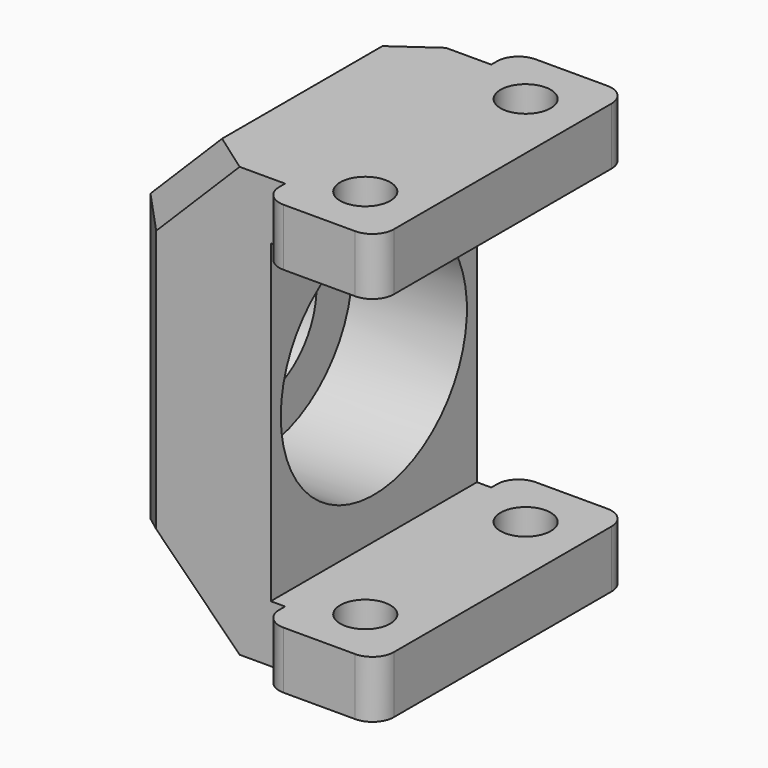
from build123d import *

# Parameters (mm, degrees)
F2_R      = 3
F2_W      = 1
F2_H      = 18
F3_DEPTH  = 4
F4_START  = 2
F2_R_2    = 1.75
F4_DEPTH  = 2
F2_W_2    = 10
F5_DEPTH  = 30
F6_START  = 26
F6_DEPTH  = 4
F7_R      = 8.125
F7_R_2    = 5
F8_DEPTH  = 10
F9_DEPTH  = 2
F10_START = 28
F10_DEPTH = 2
F11_SIZE  = 5
F12_SIZE  = 2
F13_R     = 1.5


# Not quite as in the source:
# - a feature names something its author has since deleted; it is built from what else it names


with BuildPart() as f3:
    # F2 (on Top) → F3 (new body)
    with BuildSketch(Plane.XY):
        Polygon((4, 11), (-4, 11), (-4, 9), (-4, -9), (-4, -11), (4, -11), align=None)
        with Locations((0, -7)):
            Circle(F2_R, mode=Mode.SUBTRACT)
        with Locations((0, 7)):
            Circle(F2_R, mode=Mode.SUBTRACT)
        with Locations((-4.5, 0)):
            Rectangle(F2_W, F2_H)
    extrude(amount=F3_DEPTH)

    # F2 (on Top) → F4 (join)
    with BuildSketch(Plane.XY.offset(F4_START)):
        with Locations((0, -7)):
            Circle(F2_R)
        with Locations((0, -7)):
            Circle(F2_R_2, mode=Mode.SUBTRACT)
        with Locations((0, 7)):
            Circle(F2_R)
        with Locations((0, 7)):
            Circle(F2_R_2, mode=Mode.SUBTRACT)
    extrude(amount=F4_DEPTH)

    # F2 (on Top) → F5 (join)
    with BuildSketch(Plane.XY):
        with Locations((-10, 0)):
            Rectangle(F2_W_2, F2_H)
    extrude(amount=F5_DEPTH)

    # F2 (on Top) → F6 (join)
    with BuildSketch(Plane.XY.offset(F6_START)):
        Polygon((4, 11), (-4, 11), (-4, 9), (-4, -9), (-4, -11), (4, -11), align=None)
        with Locations((0, -7)):
            Circle(F2_R, mode=Mode.SUBTRACT)
        with Locations((0, 7)):
            Circle(F2_R, mode=Mode.SUBTRACT)
        with Locations((-4.5, 0)):
            Rectangle(F2_W, F2_H)
    extrude(amount=F6_DEPTH)

    # F7 (on face) → F8 (cut)
    with BuildSketch(Plane(origin=(-15, 0, 0), x_dir=(0, -1, 0), z_dir=(-1, 0, 0))):
        with Locations((0, 15)):
            Circle(F7_R)
        with Locations((0, 15)):
            Circle(F7_R_2, mode=Mode.SUBTRACT)
        with Locations((0, 15)):
            Circle(F7_R_2)
    extrude(amount=-F8_DEPTH, mode=Mode.SUBTRACT)

    # F7 (on face) → F9 (join)
    with BuildSketch(Plane(origin=(-15, 0, 0), x_dir=(0, -1, 0), z_dir=(-1, 0, 0))):
        with Locations((0, 15)):
            Circle(F7_R)
        with Locations((0, 15)):
            Circle(F7_R_2, mode=Mode.SUBTRACT)
    extrude(amount=-F9_DEPTH)

    # F2 (on Top) → F10 (join)
    with BuildSketch(Plane.XY.offset(F10_START)):
        with Locations((0, 7)):
            Circle(F2_R)
        with Locations((0, 7)):
            Circle(F2_R_2, mode=Mode.SUBTRACT)
        with Locations((0, -7)):
            Circle(F2_R)
        with Locations((0, -7)):
            Circle(F2_R_2, mode=Mode.SUBTRACT)
    extrude(amount=F10_DEPTH)

    # F11
    f11_edges = [f3.edges().sort_by_distance(p)[0] for p in [
        (-15, 0, 0),
        (-15, 0, 30),
    ]]
    chamfer(f11_edges, length=F11_SIZE)

    # F12
    f12_edges = [f3.edges().sort_by_distance(p)[0] for p in [
        (-15, -9, 15),
        (-15, 9, 15),
        (-12.5, 9, 27.5),
        (-12.5, -9, 27.5),
        (-12.5, 9, 2.5),
        (-12.5, -9, 2.5),
    ]]
    chamfer(f12_edges, length=F12_SIZE)

    # F13
    f13_edges = [f3.edges().sort_by_distance(p)[0] for p in [
        (4, 11, 2),
        (4, -11, 2),
        (-4, -11, 2),
        (-4, 11, 2),
        (4, 11, 28),
        (-4, 11, 28),
        (-4, -11, 28),
        (4, -11, 28),
    ]]
    fillet(f13_edges, radius=F13_R)


solid = f3.part
